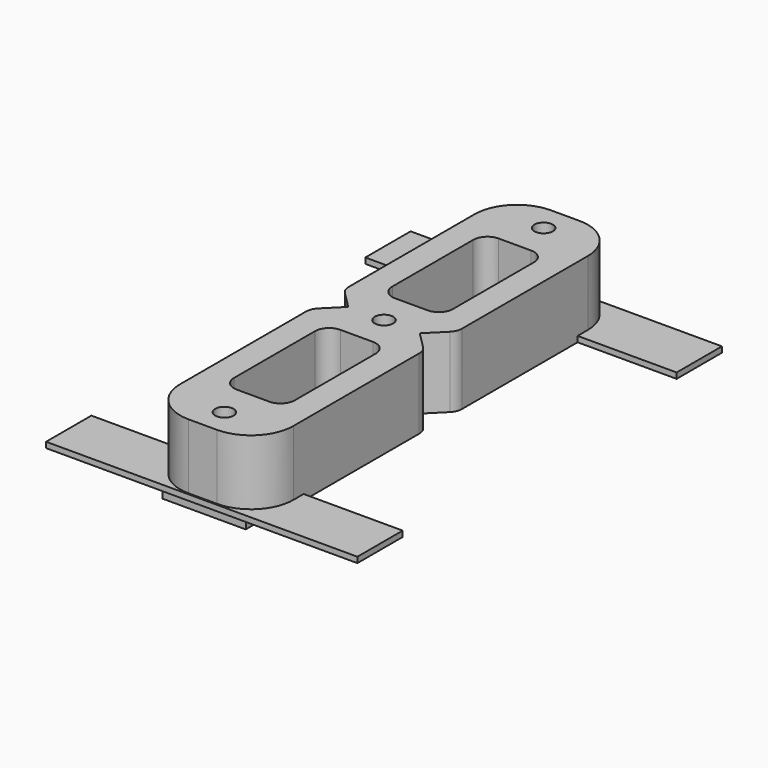
from build123d import *

# Parameters (mm, degrees)
F0_R     = 2.9
F0_W     = 29.5052044094
F0_H     = 18
F0_R_2   = 3.25
F1_DEPTH = 2
F2_DEPTH = 3
F3_R     = 3.25
F4_DEPTH = 25


# Not quite as in the source:
# - a feature names something its author has since deleted; it is built from what else it names


with BuildPart() as f1:
    # F0 (on Top) → F1 (new body)
    with BuildSketch(Plane.XY):
        Polygon((55, 80.5), (-55, 80.5), (-55, 60.5), (-11.7076300085, 60.5), (-11.7076300085, 0), (-9.1474745423, 0), (-9.1474745423, 50), (9.1474745423, 50), (9.1474745423, 0), (11.7076300085, 0), (11.7076300085, 60.5), (55, 60.5), align=None)
        with Locations((-44.5, 70.5)):
            Circle(F0_R, mode=Mode.SUBTRACT)
        with Locations((0, 70.5)):
            Rectangle(F0_W, F0_H, mode=Mode.SUBTRACT)
        with Locations((44.5, 70.5)):
            Circle(F0_R, mode=Mode.SUBTRACT)
        Polygon((-9.1474745423, 0), (-11.7076300085, 0), (-11.7076300085, -60.5), (-55, -60.5), (-55, -80.5), (55, -80.5), (55, -60.5), (11.7076300085, -60.5), (11.7076300085, -10), (11.7076300085, 0), (9.1474745423, 0), (9.1474745423, -50), (-9.1474745423, -50), align=None)
        with Locations((-44.5, -70.5)):
            Circle(F0_R, mode=Mode.SUBTRACT)
        with Locations((0, -70.5)):
            Rectangle(F0_W, F0_H, mode=Mode.SUBTRACT)
        with Locations((44.5, -70.5)):
            Circle(F0_R, mode=Mode.SUBTRACT)
        with Locations((44.5, 70.5)):
            Circle(F0_R)
        with Locations((-44.5, 70.5)):
            Circle(F0_R)
        with Locations((-44.5, -70.5)):
            Circle(F0_R)
        with Locations((44.5, -70.5)):
            Circle(F0_R)
        with Locations((0, 70.5)):
            Rectangle(F0_W, F0_H)
        with Locations((0, 70.5)):
            Circle(F0_R_2, mode=Mode.SUBTRACT)
        with Locations((0, -70.5)):
            Rectangle(F0_W, F0_H)
        with Locations((0, -70.5)):
            Circle(F0_R_2, mode=Mode.SUBTRACT)
        with BuildLine():
            Line((-9.1474745423, 50), (-9.1474745423, 0))
            Line((-9.1474745423, 0), (-3.25, 0))
            ThreePointArc((-3.25, 0), (0, 3.25), (3.25, 0))
            Line((3.25, 0), (9.1474745423, 0))
            Line((9.1474745423, 0), (9.1474745423, 50))
            Line((9.1474745423, 50), (-9.1474745423, 50))
        make_face()
        with BuildLine():
            Line((-3.25, 0), (-9.1474745423, 0))
            Line((-9.1474745423, 0), (-9.1474745423, -50))
            Line((-9.1474745423, -50), (9.1474745423, -50))
            Line((9.1474745423, -50), (9.1474745423, 0))
            Line((9.1474745423, 0), (3.25, 0))
            ThreePointArc((3.25, 0), (0, -3.25), (-3.25, 0))
        make_face()
    extrude(amount=F1_DEPTH)

    # F0 (on Top) → F2 (join)
    with BuildSketch(Plane.XY):
        with Locations((44.5, 70.5)):
            Circle(F0_R)
        with Locations((-44.5, 70.5)):
            Circle(F0_R)
        with Locations((44.5, -70.5)):
            Circle(F0_R)
        with Locations((-44.5, -70.5)):
            Circle(F0_R)
        with Locations((0, 70.5)):
            Rectangle(F0_W, F0_H)
        with Locations((0, 70.5)):
            Circle(F0_R_2, mode=Mode.SUBTRACT)
        with Locations((0, -70.5)):
            Rectangle(F0_W, F0_H)
        with Locations((0, -70.5)):
            Circle(F0_R_2, mode=Mode.SUBTRACT)
        with BuildLine():
            Line((-9.1474745423, 50), (-9.1474745423, 0))
            Line((-9.1474745423, 0), (-3.25, 0))
            ThreePointArc((-3.25, 0), (0, 3.25), (3.25, 0))
            Line((3.25, 0), (9.1474745423, 0))
            Line((9.1474745423, 0), (9.1474745423, 50))
            Line((9.1474745423, 50), (-9.1474745423, 50))
        make_face()
        with BuildLine():
            Line((-3.25, 0), (-9.1474745423, 0))
            Line((-9.1474745423, 0), (-9.1474745423, -50))
            Line((-9.1474745423, -50), (9.1474745423, -50))
            Line((9.1474745423, -50), (9.1474745423, 0))
            Line((9.1474745423, 0), (3.25, 0))
            ThreePointArc((3.25, 0), (0, -3.25), (-3.25, 0))
        make_face()
    extrude(amount=-F2_DEPTH)


with BuildPart() as f4:
    # F3 (on Top) → F4 (new body)
    with BuildSketch(Plane.XY):
        with BuildLine():
            ThreePointArc((-5, 80), (-15.6066017178, 75.6066017178), (-20, 65))
            Line((-20, 65), (-20, 9.4436440896))
            ThreePointArc((-20, 9.4436440896), (-19.6193976626, 7.5302269277), (-18.5355339059, 5.9081101836))
            Line((-18.5355339059, 5.9081101836), (-12.6274237223, 0))
            Line((-12.6274237223, 0), (-18.5355339059, -5.9081101836))
            ThreePointArc((-18.5355339059, -5.9081101836), (-19.6193976626, -7.5302269277), (-20, -9.4436440896))
            Line((-20, -9.4436440896), (-20, -65))
            ThreePointArc((-20, -65), (-15.6066017178, -75.6066017178), (-5, -80))
            Line((-5, -80), (5, -80))
            ThreePointArc((5, -80), (15.6066017178, -75.6066017178), (20, -65))
            Line((20, -65), (20, -9.4436440896))
            ThreePointArc((20, -9.4436440896), (19.6193976626, -7.5302269277), (18.5355339059, -5.9081101836))
            Line((18.5355339059, -5.9081101836), (12.6274237223, 0))
            Line((12.6274237223, 0), (18.5355339059, 5.9081101836))
            ThreePointArc((18.5355339059, 5.9081101836), (19.6193976626, 7.5302269277), (20, 9.4436440896))
            Line((20, 9.4436440896), (20, 65))
            ThreePointArc((20, 65), (15.6066017178, 75.6066017178), (5, 80))
            Line((5, 80), (-5, 80))
        make_face()
        with BuildLine():
            Line((10.7299620286, -17.0571833104), (10.7299620286, -52.8276179731))
            ThreePointArc((10.7299620286, -52.8276179731), (9.2654959345, -56.363151879), (5.7299620286, -57.8276179731))
            Line((5.7299620286, -57.8276179731), (-5.7299620286, -57.8276179731))
            ThreePointArc((-5.7299620286, -57.8276179731), (-9.2654959345, -56.363151879), (-10.7299620286, -52.8276179731))
            Line((-10.7299620286, -52.8276179731), (-10.7299620286, -17.0571833104))
            ThreePointArc((-10.7299620286, -17.0571833104), (-9.2654959345, -13.5216494045), (-5.7299620286, -12.0571833104))
            Line((-5.7299620286, -12.0571833104), (5.7299620286, -12.0571833104))
            ThreePointArc((5.7299620286, -12.0571833104), (9.2654959345, -13.5216494045), (10.7299620286, -17.0571833104))
        make_face(mode=Mode.SUBTRACT)
        with Locations((0, -70.5)):
            Circle(F3_R, mode=Mode.SUBTRACT)
        Circle(F3_R, mode=Mode.SUBTRACT)
        with BuildLine():
            ThreePointArc((-10.7299620286, 52.8276179731), (-9.2654959345, 56.363151879), (-5.7299620286, 57.8276179731))
            Line((-5.7299620286, 57.8276179731), (5.7299620286, 57.8276179731))
            ThreePointArc((5.7299620286, 57.8276179731), (9.2654959345, 56.363151879), (10.7299620286, 52.8276179731))
            Line((10.7299620286, 52.8276179731), (10.7299620286, 17.0571833104))
            ThreePointArc((10.7299620286, 17.0571833104), (9.2654959345, 13.5216494045), (5.7299620286, 12.0571833104))
            Line((5.7299620286, 12.0571833104), (-5.7299620286, 12.0571833104))
            ThreePointArc((-5.7299620286, 12.0571833104), (-9.2654959345, 13.5216494045), (-10.7299620286, 17.0571833104))
            Line((-10.7299620286, 17.0571833104), (-10.7299620286, 52.8276179731))
        make_face(mode=Mode.SUBTRACT)
        with Locations((0, 70.5)):
            Circle(F3_R, mode=Mode.SUBTRACT)
    extrude(amount=F4_DEPTH)


solid = Compound([f1.part, f4.part])
